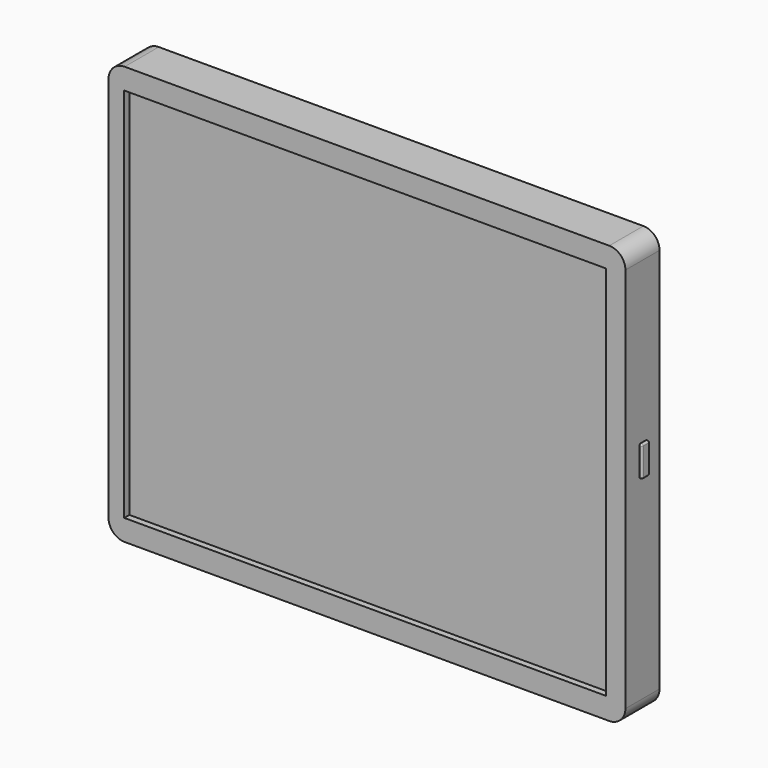
from build123d import *

# Parameters (mm, degrees)
F0_W      = 1600
F0_H      = 1295
F1_DEPTH  = 132
F2_R      = 50
F4_W      = 1491.3636445999
F4_H      = 1164.5535230637
F5_DEPTH  = 20
F7_W      = 1491.3636445999
F7_H      = 1164.5535230637
F8_DEPTH  = 100
F10_W     = 150
F10_H     = 95
F10_W_2   = 103.7647128105
F10_H_2   = 95.1176285744
F10_W_3   = 165
F10_H_3   = 190
F11_DEPTH = 100
F12_T     = -5
F13_W     = 30.2646905184
F13_H     = 95.1176509261
F14_DEPTH = 8
F15_R     = 5


# Not quite as in the source:
# - the program builds the solid bodies; features that only make, move or delete a surface that nothing else refers to are left out


with BuildPart() as f1:
    # F0 (on Front) → F1 (new body)
    with BuildSketch(Plane.XZ):
        with Locations((5.5797146633, 0)):
            Rectangle(F0_W, F0_H)
    extrude(amount=F1_DEPTH)

    # F2
    f2_edges = [f1.edges().sort_by_distance(p)[0] for p in [
        (-794.420285, -66, 647.5),
        (805.579715, -66, 647.5),
        (805.579715, -66, -647.5),
        (-794.420285, -66, -647.5),
    ]]
    fillet(f2_edges, radius=F2_R)

    # F4 (on offset) → F5 (cut)
    with BuildSketch(Plane.XZ.offset(132)):
        Rectangle(F4_W, F4_H)
    extrude(amount=-F5_DEPTH, mode=Mode.SUBTRACT)

    # F7 (on offset) → F8 (cut)
    with BuildSketch(Plane(origin=(0, 0, 0), x_dir=(-1, 0, 0), z_dir=(0, 1, 0))):
        with Locations((-8.7735056877, 2.2042393684)):
            Rectangle(F7_W, F7_H)
    extrude(amount=-F8_DEPTH, mode=Mode.SUBTRACT)

    # F10 (on offset) → F11 (join)
    with BuildSketch(Plane(origin=(0, -100, 0), x_dir=(-1, 0, 0), z_dir=(0, 1, 0))):
        with Locations((527.2952914238, -438.8382136822)):
            Rectangle(F10_W, F10_H)
        with Locations((471.1775481701, 244.2793995142)):
            Rectangle(F10_W_2, F10_H_2)
        with Locations((-473.1311607361, -343.8382136822)):
            Rectangle(F10_W_3, F10_H_3)
    extrude(amount=F11_DEPTH)

    # F12
    f12_openings = [f1.faces().sort_by_distance(p)[0] for p in [
        (-527.295291, 0, -438.838214),
        (-471.177548, 0, 244.2794),
        (473.131161, 0, -343.838214),
    ]]
    offset(amount=F12_T, openings=f12_openings, kind=Kind.INTERSECTION)

    # F13 (on face) → F14 (join)
    with BuildSketch(Plane.YZ.offset(805.5797146633)):
        with Locations((-62.757357955, 54.0441162884)):
            Rectangle(F13_W, F13_H)
    extrude(amount=F14_DEPTH)

    # F15
    f15_edges = [f1.edges().sort_by_distance(p)[0] for p in [
        (809.579715, -47.625013, 101.602942),
        (809.579715, -77.889703, 101.602942),
        (809.579715, -77.889703, 6.485291),
        (809.579715, -47.625013, 6.485291),
        (813.579715, -62.757358, 101.602942),
        (813.579715, -77.889703, 54.044116),
        (813.579715, -47.625013, 54.044116),
        (813.579715, -62.757358, 6.485291),
    ]]
    fillet(f15_edges, radius=F15_R)


solid = f1.part
